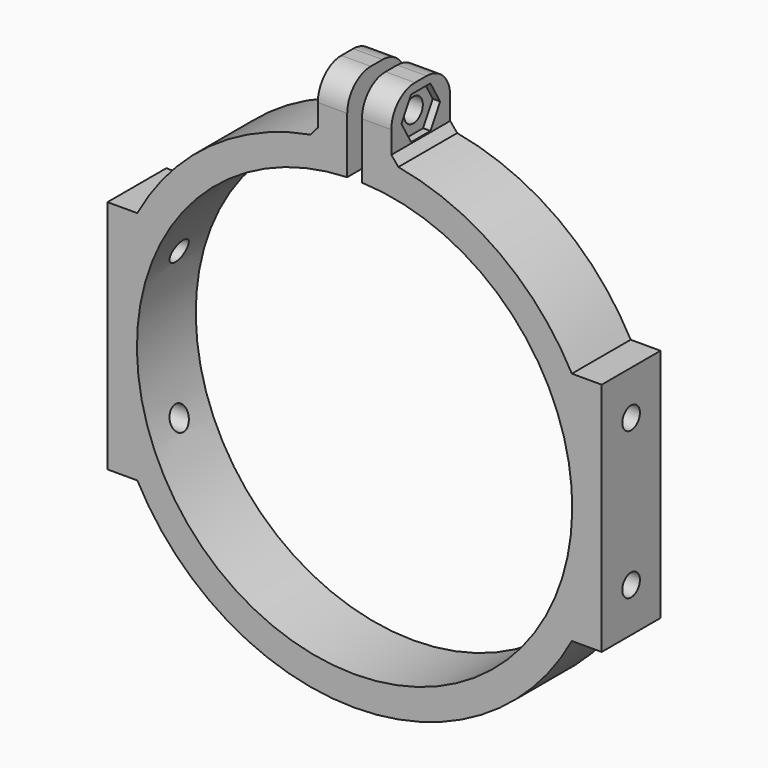
from build123d import *

# Parameters (mm, degrees)
F1_DEPTH    = 10
F2_R        = 1.5
F3_DEPTH    = 67.201
F5_DEPTH    = 1
F6_D        = 3.2
F7_R        = 4
F8_T1_DEPTH = 10


# Not quite as in the source:
# - a fillet or chamfer that OpenCascade refuses, or shapes differently, is made with other operations: its cross-section is extruded or revolved along the edge and cut away or added


with BuildPart() as f1:
    # F0 (on Front) → F1 (new body)
    with BuildSketch(Plane.XZ):
        with BuildLine():
            ThreePointArc((1, 29.5831032855), (0, -29.6), (-1, 29.5831032855))
            Line((-1, 29.5831032855), (-1, 41.225893517))
            Line((-1, 41.225893517), (-5, 41.225893517))
            Line((-5, 41.225893517), (-5, 33.225893517))
            ThreePointArc((-5, 33.225893517), (-19.3012329429, 27.503134492), (-29.5458965002, 16))
            Line((-29.5458965002, 16), (-33.6, 16))
            Line((-33.6, 16), (-33.6, -16))
            Line((-33.6, -16), (-29.5458965002, -16))
            ThreePointArc((-29.5458965002, -16), (0, -33.6), (29.5458965002, -16))
            Line((29.5458965002, -16), (33.6, -16))
            Line((33.6, -16), (33.6, 16))
            Line((33.6, 16), (29.5458965002, 16))
            ThreePointArc((29.5458965002, 16), (19.3012329429, 27.503134492), (5, 33.225893517))
            Line((5, 33.225893517), (5, 41.225893517))
            Line((5, 41.225893517), (1, 41.225893517))
            Line((1, 41.225893517), (1, 29.5831032855))
        make_face()
    extrude(amount=F1_DEPTH)

    # F2 (on face) → F3 (cut, through all)
    with BuildSketch(Plane.YZ.offset(33.6)):
        with Locations((-5, 10)):
            Circle(F2_R)
        with Locations((-5, -10)):
            Circle(F2_R)
    extrude(amount=-F3_DEPTH, mode=Mode.SUBTRACT)

    # F4 (on face) → F5 (cut)
    with BuildSketch(Plane.YZ.offset(5)):
        Polygon((-1.7091034656, 37.225893517), (-3.3545517328, 40.075893517), (-6.6454482672, 40.075893517), (-8.2908965344, 37.225893517), (-6.6454482672, 34.375893517), (-3.3545517328, 34.375893517), align=None)
    extrude(amount=-F5_DEPTH, mode=Mode.SUBTRACT)

    # F6 (through all)
    with Locations(Plane.YZ.offset(5)):
        with Locations((-5, 37.225893517)):
            Hole(F6_D / 2)

    # F7
    f7_edges = [f1.edges().sort_by_distance(p)[0] for p in [
        (3, 0, 41.225894),
        (3, -10, 41.225894),
        (-3, -10, 41.225894),
        (-3, 0, 41.225894),
    ]]
    fillet(f7_edges, radius=F7_R)

    # F8: chamfer of 1 on 2 edges, made by hand

    # F8_s2 → F8_t1 (join)
    with BuildSketch(Plane.XZ):
        with BuildLine():
            Line((4.9743446923, 34.2419704201), (5.9814730887, 33.0372447854))
            Line((5.9814730887, 33.0372447854), (5.977927959, 33.0175614916))
            ThreePointArc((5.977927959, 33.0175614916), (5.4901701774, 33.1281516451), (4.9970238095, 33.2061161994))
            Line((4.9970238095, 33.2061161994), (4.98, 33.225893517))
            ThreePointArc((4.98, 33.225893517), (4.98, 33.7339319685), (4.9543446923, 34.2419704201))
            Line((4.9543446923, 34.2419704201), (4.9743446923, 34.2419704201))
        make_face()
        with BuildLine():
            Line((-4.9743446923, 34.2419704201), (-5.9814730887, 33.0372447854))
            Line((-5.9814730887, 33.0372447854), (-5.977927959, 33.0175614916))
            ThreePointArc((-5.977927959, 33.0175614916), (-5.4901701774, 33.1281516451), (-4.9970238095, 33.2061161994))
            Line((-4.9970238095, 33.2061161994), (-4.98, 33.225893517))
            ThreePointArc((-4.98, 33.225893517), (-4.98, 33.7339319685), (-4.9543446923, 34.2419704201))
            Line((-4.9543446923, 34.2419704201), (-4.9743446923, 34.2419704201))
        make_face()
    extrude(amount=F8_T1_DEPTH)


solid = f1.part
